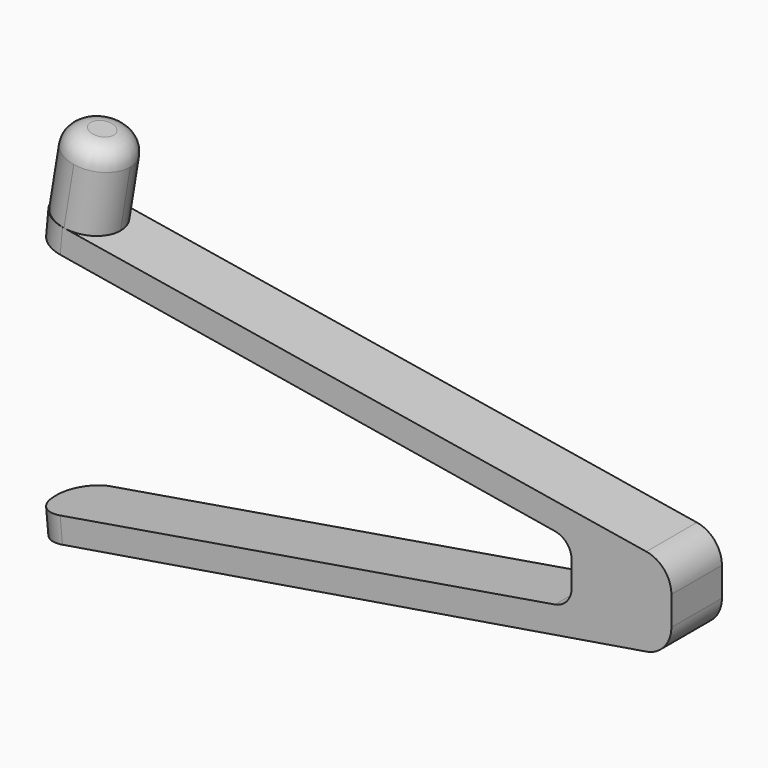
from build123d import *

# Parameters (mm, degrees)
F1_DEPTH = 6.33
F2_R     = 2
F3_R     = 3
F5_DEPTH = 8
F7_R     = 3


# Not quite as in the source:
# - a fillet or chamfer that OpenCascade refuses, or shapes differently, is made with other operations: its cross-section is extruded or revolved along the edge and cut away or added


with BuildPart() as f1:
    # F0 (on Front) → F1 (new body)
    with BuildSketch(Plane.XZ):
        Polygon((34, 4), (-30, 14.5), (-30.2323504967, 12), (24, 2.9564342819), (24, -2.9564342819), (-30.2323504967, -12), (-30, -14.5), (34, -4), align=None)
    extrude(amount=F1_DEPTH)

    # F2
    f2_edges = [f1.edges().sort_by_distance(p)[0] for p in [
        (24, -3.165, -2.956434),
        (24, -3.165, 2.956434),
    ]]
    fillet(f2_edges, radius=F2_R)

    # F3
    f3_edges = [f1.edges().sort_by_distance(p)[0] for p in [
        (34, -3.165, 4),
        (34, -3.165, -4),
    ]]
    fillet(f3_edges, radius=F3_R)

    # F4 (on face) → F5 (join)
    with BuildSketch(Plane(origin=(1.5302228826, 0, 9.3270728083), x_dir=(0.9868074809, 0, -0.1618981023), z_dir=(0.1618981023, 0, 0.9868074809))):
        with BuildLine():
            ThreePointArc((-28.7867469125, -6.33), (-26.54875395, -5.4029929625), (-25.6217469125, -3.165))
            ThreePointArc((-25.6217469125, -3.165), (-26.54875395, -0.9270070375), (-28.7867469125, 0))
            ThreePointArc((-28.7867469125, 0), (-31.0247398749, -0.9270070375), (-31.9517469125, -3.165))
            ThreePointArc((-31.9517469125, -3.165), (-31.0247398749, -5.4029929625), (-28.7867469125, -6.33))
        make_face()
    extrude(amount=F5_DEPTH)

    # F6: fillet of radius 2 on 1 edges, made by hand

    # F6_s1 → F6_t2 (revolve, cut)
    with BuildSketch(Plane.XZ.offset(3.165)):
        with BuildLine():
            ThreePointArc((-29.0286113859, 20.4208448857), (-28.221594455, 21.7215636961), (-26.7312002194, 22.0706636429))
            Line((-26.7312002194, 22.0706636429), (-28.7048151813, 22.3944598476))
            Line((-28.7048151813, 22.3944598476), (-29.0286113859, 20.4208448857))
        make_face()
    revolve(axis=Axis((-25.581569504, -3.165, 21.8820523537), (-0.1618981023, 0, -0.9868074809)), mode=Mode.SUBTRACT)

    # F7
    f7_edges = [f1.edges().sort_by_distance(p)[0] for p in [
        (-30.116175, 0, 13.25),
        (-30.116175, -6.33, 13.25),
        (-30.116175, 0, -13.25),
        (-30.116175, -6.33, -13.25),
    ]]
    fillet(f7_edges, radius=F7_R)


solid = f1.part
